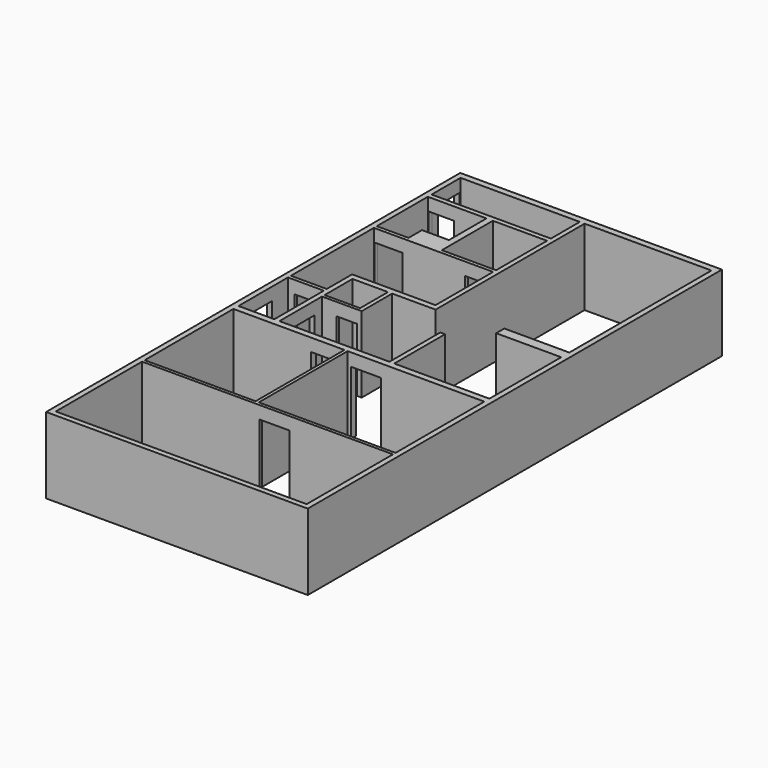
from build123d import *

# Parameters (mm, degrees)
F0_W     = 1130
F0_H     = 1950
F0_W_2   = 1120
F0_H_2   = 1100
F0_W_3   = 3760
F0_H_3   = 1140
F0_W_4   = 1710
F0_H_4   = 2010
F0_W_5   = 850
F0_H_5   = 530
F1_DEPTH = 2400
F3_START = -400
F2_W     = 170
F2_H     = 850
F2_W_2   = 800
F2_H_2   = 150
F2_W_3   = 880
F2_H_3   = 115
F2_W_4   = 870
F2_W_5   = 850
F2_H_4   = 880
F2_W_6   = 650
F2_H_5   = 100
F2_W_7   = 160
F2_W_8   = 950
F2_H_6   = 200
F3_DEPTH = 2000


# Not quite as in the source:
# - a feature names something its author has since deleted; it is built from what else it names


with BuildPart() as f1:
    # F0 (on Top) → F1 (new body)
    with BuildSketch(Plane.XY):
        Polygon((4125, 0), (-4125, 0), (-4125, -9150), (-3955, -9150), (-455, -9150), (-355, -9150), (3955, -9150), (4125, -9150), align=None)
        with Locations((-3390, -7975)):
            Rectangle(F0_W, F0_H, mode=Mode.SUBTRACT)
        with Locations((-2105, -6620)):
            Rectangle(F0_W_2, F0_H_2, mode=Mode.SUBTRACT)
        Polygon((-3955, -5885), (-3955, -3615), (-195, -3615), (-195, -5885), (-2825, -5885), (-2825, -6885), (-3955, -6885), align=None, mode=Mode.SUBTRACT)
        Polygon((-3955, -3500), (-3955, -1490), (-2105, -1490), (-2105, -2970), (-2105, -3500), (-2955, -3500), align=None, mode=Mode.SUBTRACT)
        with Locations((-2075, -770)):
            Rectangle(F0_W_3, F0_H_3, mode=Mode.SUBTRACT)
        with Locations((-1050, -2495)):
            Rectangle(F0_W_4, F0_H_4, mode=Mode.SUBTRACT)
        Polygon((-45, -6070), (-45, -200), (3955, -200), (3955, -5800), (1905, -5800), (1905, -6120), (3955, -6120), (3955, -8950), (955, -8950), (955, -6950), (805, -6950), (805, -8950), (-2665, -8950), (-2665, -7270), (-1415, -7270), (-1415, -6070), align=None, mode=Mode.SUBTRACT)
        with Locations((-2530, -3235)):
            Rectangle(F0_W_5, F0_H_5)
        Polygon((-355, -9150), (-455, -9150), (-455, -12650), (-3955, -12650), (-3955, -12750), (-355, -12750), (3955, -12750), (3955, -12650), (-355, -12650), align=None)
        Polygon((-3955, -9150), (-4125, -9150), (-4125, -16320), (4125, -16320), (4125, -9150), (3955, -9150), (3955, -12650), (3955, -12750), (3955, -16150), (-3955, -16150), (-3955, -12750), (-3955, -12650), align=None)
    extrude(amount=F1_DEPTH)

    # F2 (on face) → F3 (cut)
    with BuildSketch(Plane.XY.offset(2400).offset(F3_START)):
        with Locations((-4040, -665)):
            Rectangle(F2_W, F2_H)
        with Locations((-3535, -1415)):
            Rectangle(F2_W_2, F2_H_2)
        with Locations((-3495, -3557.5)):
            Rectangle(F2_W_3, F2_H_3)
        with Locations((-640, -3557.5)):
            Rectangle(F2_W_4, F2_H_3)
        with Locations((-3330, -6942.5)):
            Rectangle(F2_W_5, F2_H_3)
        with Locations((-4040, -8060)):
            Rectangle(F2_W, F2_H_4)
        with Locations((-1890, -7220)):
            Rectangle(F2_W_6, F2_H_5)
        with Locations((-2745, -8010)):
            Rectangle(F2_W_7, F2_H_4)
        with Locations((-1030, -9050)):
            Rectangle(F2_W_8, F2_H_6)
        with Locations((220, -9050)):
            Rectangle(F2_W_8, F2_H_6)
        with Locations((220, -12700)):
            Rectangle(F2_W_8, F2_H_5)
    extrude(amount=-F3_DEPTH, mode=Mode.SUBTRACT)


solid = f1.part
